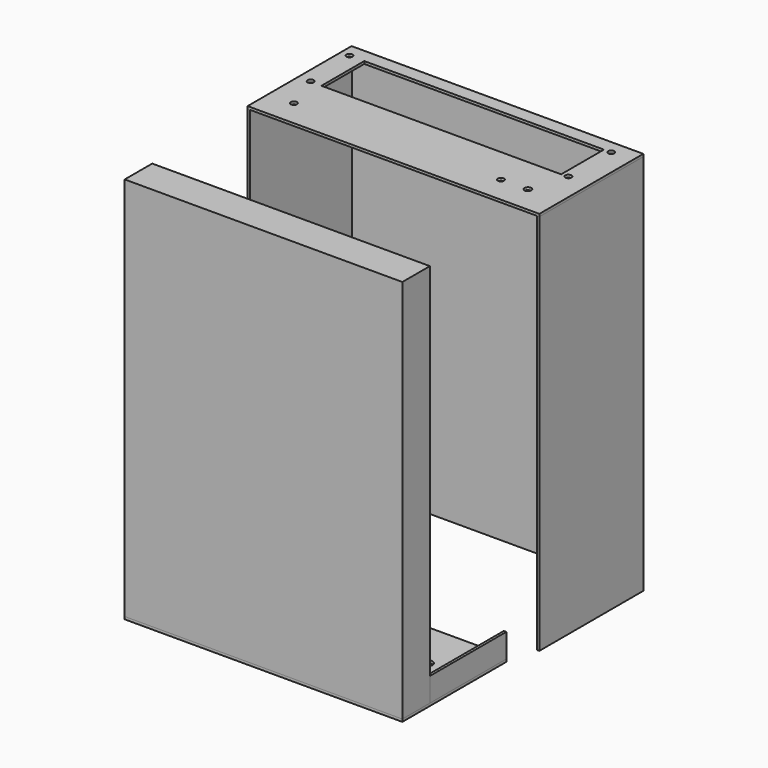
from build123d import *

# Parameters (mm, degrees)
F1_DEPTH  = 120
F0_W      = 90
F0_H      = 40
F0_R      = 0.9725861443
F0_R_2    = 1.0729216039
F0_W_2    = 75.2601372078
F0_H_2    = 16.8051975779
F2_DEPTH  = 0.8
F4_W      = 0.8
F4_H      = 30
F5_DEPTH  = 0.8
F6_DEPTH  = 120
F7_DEPTH  = 7.5
F8_W      = 85.5735123101
F8_H      = 10
F9_DEPTH  = 0.8
F4_R      = 1.6
F10_DEPTH = 0.8


with BuildPart() as f1:
    # F0 (on Top) → F1 (new body)
    with BuildSketch(Plane.XY):
        Polygon((0, -40), (0, 0), (90, 0), (90, -40), (90.8, -40), (90.8, 0.8), (-0.8, 0.8), (-0.8, -40), align=None)
    extrude(amount=-F1_DEPTH)


with BuildPart() as f2:
    # F0 (on Top) → F2 (new body)
    with BuildSketch(Plane.XY):
        Polygon((0, -40), (0, 0), (90, 0), (90, -40), (90.8, -40), (90.8, 0.8), (-0.8, 0.8), (-0.8, -40), align=None)
        with Locations((45, -20)):
            Rectangle(F0_W, F0_H)
        with Locations((7.0911361836, -31.7015498877)):
            Circle(F0_R, mode=Mode.SUBTRACT)
        with Locations((3.0214360449, -20.0629532337)):
            Circle(F0_R, mode=Mode.SUBTRACT)
        with Locations((72.0911361836, -31.7015498877)):
            Circle(F0_R, mode=Mode.SUBTRACT)
        with Locations((80.4413557053, -31.5211080015)):
            Circle(F0_R_2, mode=Mode.SUBTRACT)
        with Locations((83.9599892497, -20.0629532337)):
            Circle(F0_R, mode=Mode.SUBTRACT)
        with Locations((44.2290580831, -11.8647648487)):
            Rectangle(F0_W_2, F0_H_2, mode=Mode.SUBTRACT)
        with Locations((1.9526774995, -3.4621660598)):
            Circle(F0_R, mode=Mode.SUBTRACT)
        with Locations((84.1404348612, -3.4621660598)):
            Circle(F0_R, mode=Mode.SUBTRACT)
    extrude(amount=F2_DEPTH)


with BuildPart() as f5:
    # F4 (on offset) → F5 (new body)
    with BuildSketch(Plane.XY.offset(-120)):
        with Locations((0.4, -63.4340933131)):
            Rectangle(F4_W, F4_H)
        Polygon((0.8, -78.4340933131), (0, -78.4340933131), (0, -89.2340933131), (87.1735123101, -89.2340933131), (87.1735123101, -78.4340933131), (86.3735123101, -78.4340933131), (86.3735123101, -88.4340933131), (0.8, -88.4340933131), align=None)
        with Locations((86.7735123101, -63.4340933131)):
            Rectangle(F4_W, F4_H)
    extrude(amount=-F5_DEPTH)


with BuildPart() as f6:
    # F4 (on offset) → F6 (new body)
    with BuildSketch(Plane.XY.offset(-120)):
        Polygon((0.8, -78.4340933131), (0, -78.4340933131), (0, -89.2340933131), (87.1735123101, -89.2340933131), (87.1735123101, -78.4340933131), (86.3735123101, -78.4340933131), (86.3735123101, -88.4340933131), (0.8, -88.4340933131), align=None)
    extrude(amount=F6_DEPTH)

    # F8 (on face) → F9 (join)
    with BuildSketch(Plane.XY):
        Polygon((0, -78.4340933131), (0, -89.2340933131), (87.1735123101, -89.2340933131), (87.1735123101, -78.4340933131), (86.3735123101, -78.4340933131), (86.3735123101, -88.4340933131), (0.8, -88.4340933131), (0.8, -78.4340933131), align=None)
        with Locations((43.586756155, -83.4340933131)):
            Rectangle(F8_W, F8_H)
    extrude(amount=F9_DEPTH)


with BuildPart() as f7:
    # F4 (on offset) → F7 (new body)
    with BuildSketch(Plane.XY.offset(-120)):
        with Locations((86.7735123101, -63.4340933131)):
            Rectangle(F4_W, F4_H)
    extrude(amount=F7_DEPTH)


with BuildPart() as f7b:
    # F4 (on offset) → F7, piece 2 (new body)
    with BuildSketch(Plane.XY.offset(-120)):
        with Locations((0.4, -63.4340933131)):
            Rectangle(F4_W, F4_H)
    extrude(amount=F7_DEPTH)


with BuildPart() as f10:
    # F4 (on offset) → F10 (new body)
    with BuildSketch(Plane.XY.offset(-120)):
        Polygon((86.3735123101, -48.4340933131), (0.8, -48.4340933131), (0.8, -78.4340933131), (0.8, -88.4340933131), (86.3735123101, -88.4340933131), (86.3735123101, -78.4340933131), align=None)
        with Locations((8.708095178, -63.4340933131)):
            Circle(F4_R, mode=Mode.SUBTRACT)
        with Locations((74.4362887124, -63.4340933131)):
            Circle(F4_R, mode=Mode.SUBTRACT)
    extrude(amount=F10_DEPTH)


solid = Compound([f1.part, f2.part, f5.part, f6.part, f7.part, f7b.part, f10.part])
